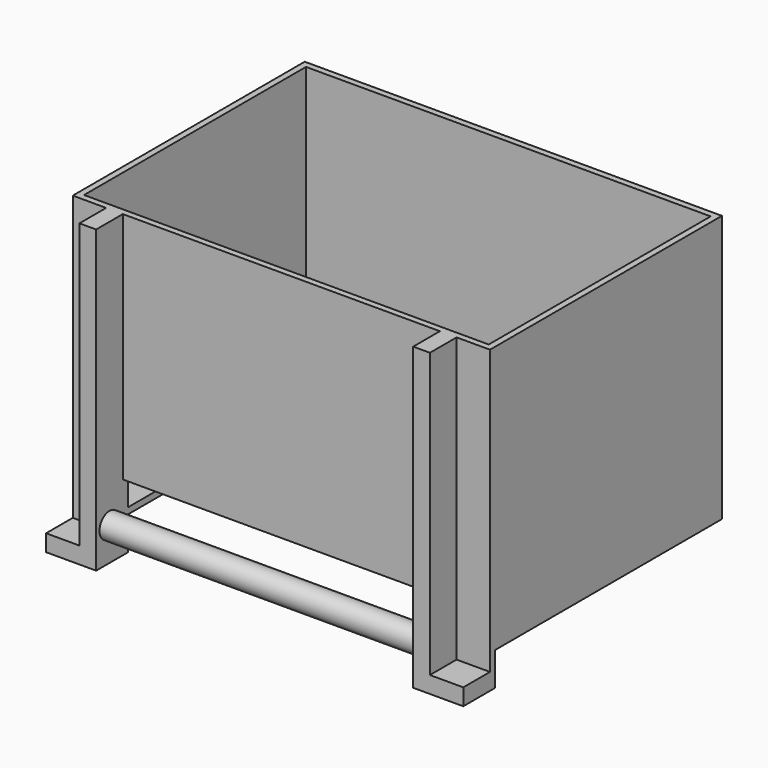
from build123d import *

# Parameters (mm, degrees)
F0_W      = 25.4
F0_H      = 50.8
F1_DEPTH  = 457.2
F2_W      = 50.8
F2_H      = 25.4
F3_DEPTH  = 50.8
F4_R      = 19.05
F5_DEPTH  = 241.3
F7_W      = 50.8
F7_H      = 431.8
F8_DEPTH  = 9.525
F11_DEPTH = 9.525
F12_W     = 9.525
F12_H     = 406.4
F13_DEPTH = 431.8
F14_W     = 615.95
F14_H     = 9.525
F15_DEPTH = 396.875


# Not quite as in the source:
# - a feature names something its author has since deleted; it is built from what else it names


with BuildPart() as f1:
    # F0 (on Top) → F1 (new body)
    with BuildSketch(Plane.XY):
        with Locations((-254, 0)):
            Rectangle(F0_W, F0_H)
    extrude(amount=F1_DEPTH)

    # F2 (on face) → F3 (join)
    with BuildSketch(Plane(origin=(-266.7, 0, 0), x_dir=(0, -1, 0), z_dir=(-1, 0, 0))):
        with Locations((0, 12.7)):
            Rectangle(F2_W, F2_H)
    extrude(amount=F3_DEPTH)

    # F4 (on face) → F5 (join)
    with BuildSketch(Plane.YZ.offset(-241.3)):
        with Locations((0, 50.8)):
            Circle(F4_R)
    extrude(amount=F5_DEPTH)

    # F6: F1 across plane


with BuildPart() as f1_1:
    add(f1.part)
    add(f1.part.mirror(Plane.YZ))

    # F7 (on face) → F8 (join)
    with BuildSketch(Plane(origin=(0, 25.4, 0), x_dir=(-1, 0, 0), z_dir=(0, 1, 0))):
        Polygon((241.3, 0), (317.5, 0), (317.5, 25.4), (266.7, 25.4), (266.7, 457.2), (241.3, 457.2), (241.3, 101.6), align=None)
        with Locations((292.1, 241.3)):
            Rectangle(F7_W, F7_H)
        Polygon((0, 101.6), (241.3, 101.6), (241.3, 457.2), (0, 457.2), (-241.3, 457.2), (-241.3, 101.6), align=None)
        Polygon((-241.3, 0), (-241.3, 101.6), (-241.3, 457.2), (-317.5, 457.2), (-317.5, 0), align=None)
    extrude(amount=F8_DEPTH)

    # F10 (on offset) → F11 (join)
    with BuildSketch(Plane.XY.offset(50.8)):
        Polygon((-307.975, 34.925), (-241.3, 34.925), (-241.3, 161.925), (241.3, 161.925), (241.3, 34.925), (307.975, 34.925), (307.975, 466.725), (-307.975, 466.725), align=None)
    extrude(amount=F11_DEPTH)

    # F12 (on face) → F13 (join)
    with BuildSketch(Plane(origin=(0, 34.925, 0), x_dir=(-1, 0, 0), z_dir=(0, 1, 0))):
        with Locations((-312.7375, 254)):
            Rectangle(F12_W, F12_H)
        with Locations((312.7375, 254)):
            Rectangle(F12_W, F12_H)
    extrude(amount=F13_DEPTH)

    # F14 (on face) → F15 (join, through all)
    with BuildSketch(Plane.XY.offset(60.325)):
        with Locations((0, 461.9625)):
            Rectangle(F14_W, F14_H)
    extrude(amount=F15_DEPTH)


solid = f1_1.part
